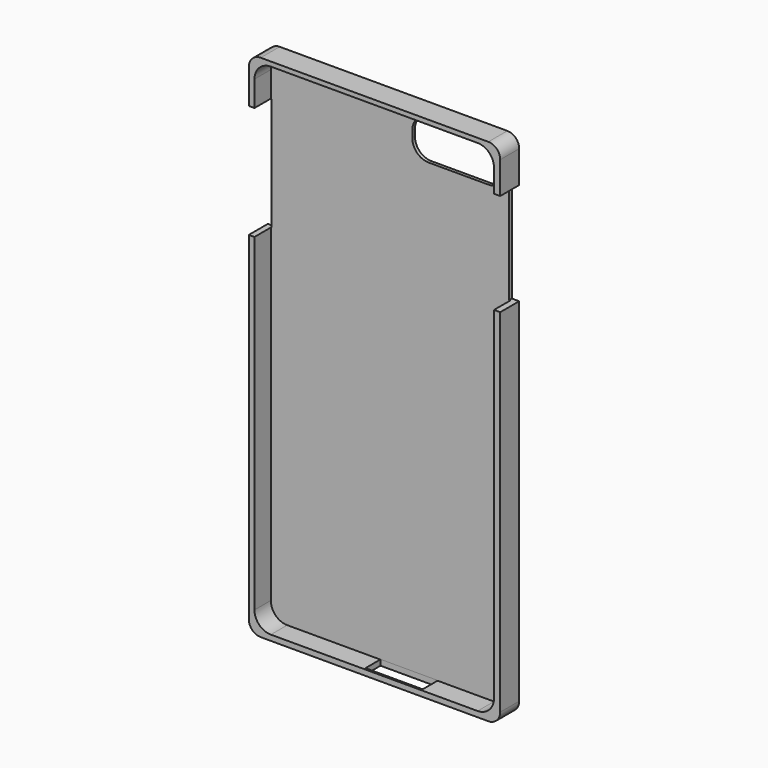
from build123d import *

# Parameters (mm, degrees)
F0_W          = 77.978
F0_H          = 158.242
F1_DEPTH      = 7.366
F3_W          = 74.3046607822
F3_H          = 155.1272720098
F4_DEPTH      = 6.35
F5_R          = 3.6792614691
F6_R          = 3.683
F7_R          = 5.08
F8_W          = 17.7591592073
F8_H          = 5.8461832232
F9_DEPTH      = 1.8034
F10_W         = 28.6683542944
F10_H         = 12.237651214
F12_DEPTH     = 25.4
F13_R         = 5.08
F14_W         = 7.366
F14_H         = 31.7207016051
F15_DEPTH     = 2.286
F16_W         = 7.366
F16_H         = 35.1969487965
F17_DEPTH     = 2.032
F18_TEXT_SIZE = 48.3377936366
F19_DEPTH     = 2.032


# Not quite as in the source:
# - Text() gives the source's letters only with a copy of the font that has no kerning and outlines rounded to 1/6400 em; it was checked with that copy


with BuildPart() as f1:
    # F0 (on Front) → F1 (new body)
    with BuildSketch(Plane.XZ):
        with Locations((-6.6413842366, 8.3520337939)):
            Rectangle(F0_W, F0_H)
    extrude(amount=F1_DEPTH)

    # F3 (on face) → F4 (cut)
    with BuildSketch(Plane.XZ.offset(7.366)):
        with Locations((-6.7260796204, 8.5133388638)):
            Rectangle(F3_W, F3_H)
    extrude(amount=-F4_DEPTH, mode=Mode.SUBTRACT)

    # F5
    f5_edges = [f1.edges().sort_by_distance(p)[0] for p in [
        (32.347616, -3.683, 87.473034),
    ]]
    fillet(f5_edges, radius=F5_R)

    # F6
    f6_edges = [f1.edges().sort_by_distance(p)[0] for p in [
        (32.347616, -3.683, -70.768966),
        (-45.630384, -3.683, -70.768966),
        (-45.630384, -3.683, 87.473034),
    ]]
    fillet(f6_edges, radius=F6_R)

    # F7
    f7_edges = [f1.edges().sort_by_distance(p)[0] for p in [
        (-43.87841, -4.191, 86.076975),
        (30.426251, -4.191, 86.076975),
        (-43.87841, -4.191, -69.050297),
        (30.426251, -4.191, -69.050297),
    ]]
    fillet(f7_edges, radius=F7_R)

    # F8 (on face) → F9 (cut)
    with BuildSketch(Plane(origin=(0, 0, -70.7689662061), x_dir=(1, 0, 0), z_dir=(0, 0, -1))):
        with Locations((-1.0431380942, 3.8613092911)):
            Rectangle(F8_W, F8_H)
    extrude(amount=-F9_DEPTH, mode=Mode.SUBTRACT)

    # F10 (on face) → F12 (cut)
    with BuildSketch(Plane(origin=(0, 0, 0), x_dir=(-1, 0, 0), z_dir=(0, 1, 0))):
        with Locations((-14.3341771472, 77.6749467179)):
            Rectangle(F10_W, F10_H)
    extrude(amount=-F12_DEPTH, mode=Mode.SUBTRACT)

    # F13
    f13_edges = [f1.edges().sort_by_distance(p)[0] for p in [
        (0, -0.508, 83.793772),
        (28.668354, -0.508, 71.556121),
        (28.668354, -0.508, 83.793772),
        (0, -0.508, 71.556121),
    ]]
    fillet(f13_edges, radius=F13_R)

    # F14 (on face) → F15 (cut)
    with BuildSketch(Plane.YZ.offset(32.3476157634)):
        with Locations((-3.683, 57.9974036664)):
            Rectangle(F14_W, F14_H)
    extrude(amount=-F15_DEPTH, mode=Mode.SUBTRACT)

    # F16 (on face) → F17 (cut)
    with BuildSketch(Plane(origin=(-45.6303842366, 0, 0), x_dir=(0, -1, 0), z_dir=(-1, 0, 0))):
        with Locations((3.683, 55.4985608906)):
            Rectangle(F16_W, F16_H)
    extrude(amount=-F17_DEPTH, mode=Mode.SUBTRACT)

    # F18 (on face) → F19 (join)
    with BuildSketch(Plane(origin=(0, 0, 0), x_dir=(-1, 0, 0), z_dir=(0, 1, 0))):
        with Locations(Location((21.8988643366, -57.5862413753), (0, 0, 90))):
            Text('3DBK', F18_TEXT_SIZE, font='Open Sans', text_align=(TextAlign.LEFT, TextAlign.BOTTOM))
    extrude(amount=F19_DEPTH)


solid = f1.part
